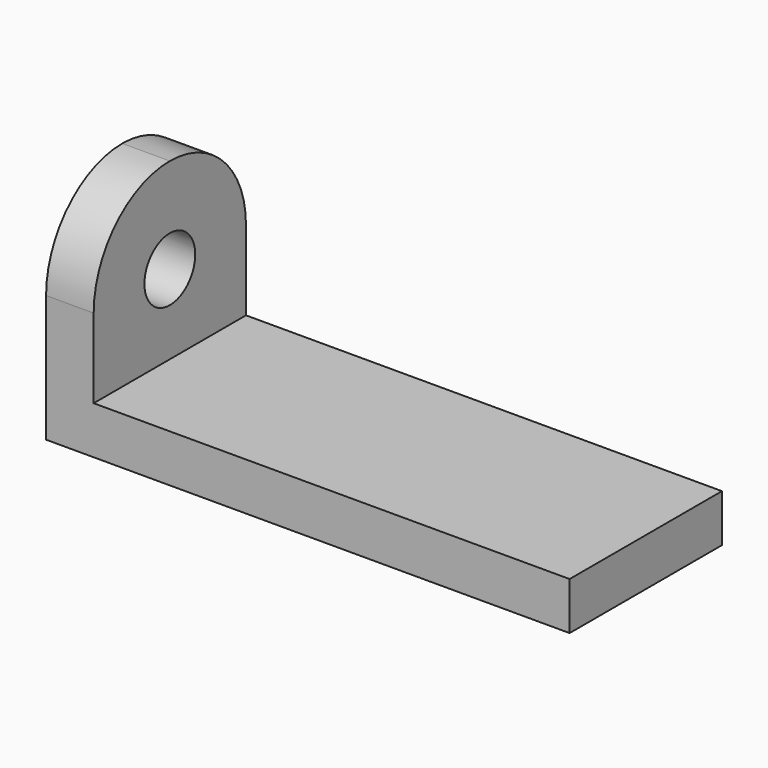
from build123d import *

# Parameters (mm, degrees)
F0_W     = 167.64
F0_H     = 60.96
F1_DEPTH = 15.24
F2_W     = 15.24
F2_H     = 60.96
F3_DEPTH = 55.88
F4_R     = 30.47999
F5_R     = 10.16
F6_DEPTH = 15.24


# Not quite as in the source:
# - a fillet or chamfer is up to 0.001 mm smaller than in the source, because OpenCascade refuses the exact size


with BuildPart() as f1:
    # F0 (on Top) → F1 (new body)
    with BuildSketch(Plane.XY):
        with Locations((50.7921350074, 13.222941007)):
            Rectangle(F0_W, F0_H)
    extrude(amount=F1_DEPTH)

    # F2 (on face) → F3 (join)
    with BuildSketch(Plane.XY.offset(15.24)):
        with Locations((-25.4078649926, 13.222941007)):
            Rectangle(F2_W, F2_H)
    extrude(amount=F3_DEPTH)

    # F4 (radius 30.48 in the source; OpenCascade refuses exactly that, so slightly less here)
    f4_edges = [f1.edges().sort_by_distance(p)[0] for p in [
        (-25.407865, -17.257059, 71.12),
        (-25.407865, 43.702941, 71.12),
    ]]
    fillet(f4_edges, radius=F4_R)

    # F5 (on face) → F6 (cut)
    with BuildSketch(Plane(origin=(-33.0278649926, 0, 0), x_dir=(0, -1, 0), z_dir=(-1, 0, 0))):
        with Locations((-13.222941007, 40.64)):
            Circle(F5_R)
    extrude(amount=-F6_DEPTH, mode=Mode.SUBTRACT)


solid = f1.part
